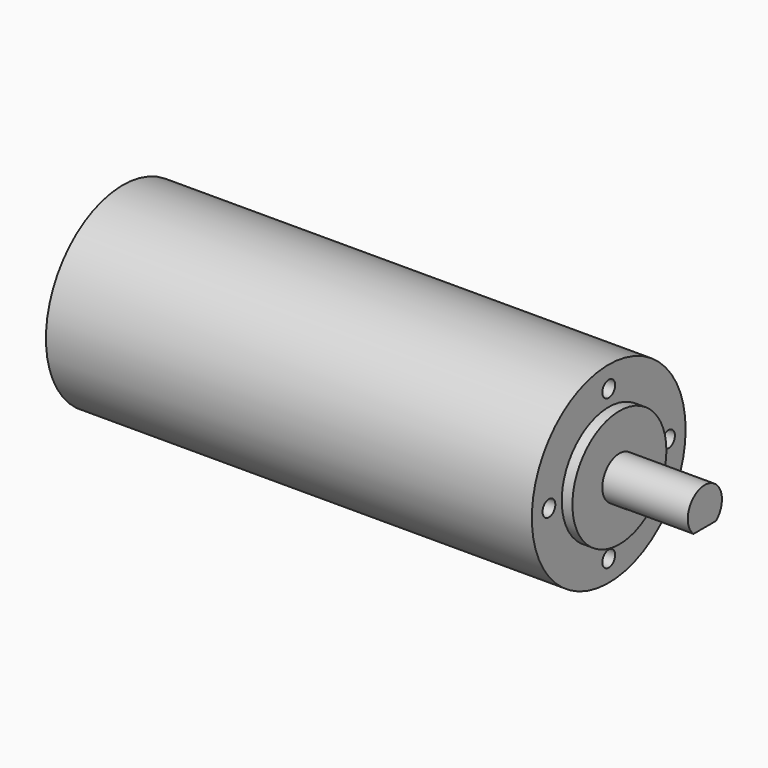
from build123d import *

# Parameters (mm, degrees)
F0_R            = 18
F1_DEPTH        = 91
F2_R            = 11
F3_DEPTH        = 2
F4_R            = 4
F5_DEPTH        = 18
F6_R            = 1.5
F7_DEPTH        = 5
F7_COPIES_COUNT = 4
F9_START        = 5
F8_W            = 60
F8_H            = 10
F9_DEPTH        = 20


# Not quite as in the source:
# - a pattern or mirror of a feature is missing from the dataset's text; its kind, count and spacing are read off the source's solid


with BuildPart() as f1:
    # F0 (on Right) → F1 (new body)
    with BuildSketch(Plane.YZ):
        Circle(F0_R)
    extrude(amount=-F1_DEPTH)

    # F2 (on Right) → F3 (join)
    with BuildSketch(Plane.YZ):
        Circle(F2_R)
    extrude(amount=F3_DEPTH)

    # F4 (on Right) → F5 (join)
    with BuildSketch(Plane.YZ):
        Circle(F4_R)
    extrude(amount=F5_DEPTH)

    # F6 (on Right) → F7 (cut)
    with BuildSketch(Plane.YZ):
        with Locations((14, 0)):
            Circle(F6_R)
    f7 = extrude(amount=-F7_DEPTH, mode=Mode.SUBTRACT)

    # F7_copies: F7 ×4 about axis
    f7_copies_axis = Axis((0, 0, 0), (1, 0, 0))
    for i in range(1, F7_COPIES_COUNT):
        add(f7.rotate(f7_copies_axis, i * 360 / F7_COPIES_COUNT), mode=Mode.SUBTRACT)

    # F8 (on Right) → F9 (cut)
    with BuildSketch(Plane.YZ.offset(F9_START)):
        with Locations((0, -8)):
            Rectangle(F8_W, F8_H)
    extrude(amount=F9_DEPTH, mode=Mode.SUBTRACT)


solid = f1.part
